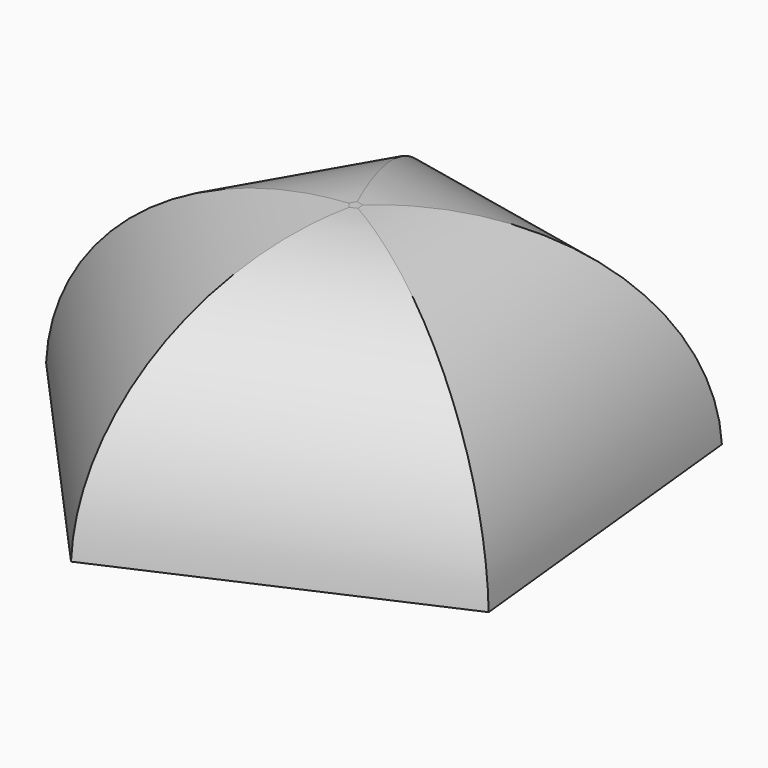
from build123d import *

# Parameters (mm, degrees)
F1_DEPTH    = 30
F2_T1_DEPTH = 201.5265861528
F2_T3_DEPTH = 201.5265861528
F2_T5_DEPTH = 201.5265861528
F2_T7_DEPTH = 201.5265861528
F2_T9_DEPTH = 201.5265861528


# Not quite as in the source:
# - a fillet or chamfer that OpenCascade refuses, or shapes differently, is made with other operations: its cross-section is extruded or revolved along the edge and cut away or added


with BuildPart() as f1:
    # F0 (on Top) → F1 (new body)
    with BuildSketch(Plane.XY):
        Polygon((-15.9371768066, 35.8527074811), (-39.0228095523, -4.0780599472), (-8.1802458333, -38.3730871366), (33.967139591, -19.6378121565), (29.1730926011, 26.2362517592), align=None)
    extrude(amount=F1_DEPTH)

    # F2: fillet of radius 31.1 on 5 edges, made by hand

    # F2_s2 → F2_t1 (cut)
    with BuildSketch(Plane(origin=(50.4334024594, 87.2336698068, 0), x_dir=(0, 0, 1), z_dir=(-0.5005136386, -0.8657286512, 0))):
        with BuildLine():
            ThreePointArc((0, 31.7420396575), (21.2765502256, 22.2601101881), (30, 0.6614991217))
            Line((30, 0.6614991217), (30, 31.7420396575))
            Line((30, 31.7420396575), (0, 31.7420396575))
        make_face()
    extrude(amount=F2_T1_DEPTH, mode=Mode.SUBTRACT)

    # F2_s4 → F2_t3 (cut)
    with BuildSketch(Plane(origin=(-67.379371666, 74.9217025, 0), x_dir=(0, 0, 1), z_dir=(0.6686896548, -0.7435416233, 0))):
        with BuildLine():
            ThreePointArc((0, 31.7420396575), (21.2765502256, 22.2601101881), (30, 0.6614991217))
            Line((30, 0.6614991217), (30, 31.7420396575))
            Line((30, 31.7420396575), (0, 31.7420396575))
        make_face()
    extrude(amount=F2_T3_DEPTH, mode=Mode.SUBTRACT)

    # F2_s6 → F2_t5 (cut)
    with BuildSketch(Plane(origin=(-92.0761442896, -40.9295111669, 0), x_dir=(0, 0, 1), z_dir=(0.9137865732, 0.406194656, 0))):
        with BuildLine():
            ThreePointArc((0, 31.7420396575), (21.2765502256, 22.2601101881), (30, 0.6614991217))
            Line((30, 0.6614991217), (30, 31.7420396575))
            Line((30, 31.7420396575), (0, 31.7420396575))
        make_face()
    extrude(amount=F2_T5_DEPTH, mode=Mode.SUBTRACT)

    # F2_s8 → F2_t7 (cut)
    with BuildSketch(Plane(origin=(10.473184942, -100.217531544, 0), x_dir=(0, 0, 1), z_dir=(-0.1039384941, 0.9945837267, 0))):
        with BuildLine():
            ThreePointArc((0, 31.7420396575), (21.2765502256, 22.2601101881), (30, 0.6614991217))
            Line((30, 0.6614991217), (30, 31.7420396575))
            Line((30, 31.7420396575), (0, 31.7420396575))
        make_face()
    extrude(amount=F2_T7_DEPTH, mode=Mode.SUBTRACT)

    # F2_s10 → F2_t9 (cut)
    with BuildSketch(Plane(origin=(98.5489285542, -21.0083295959, 0), x_dir=(0, 0, 1), z_dir=(-0.9780240953, 0.2084918918, 0))):
        with BuildLine():
            ThreePointArc((0, 31.7420396575), (21.2765502256, 22.2601101881), (30, 0.6614991217))
            Line((30, 0.6614991217), (30, 31.7420396575))
            Line((30, 31.7420396575), (0, 31.7420396575))
        make_face()
    extrude(amount=F2_T9_DEPTH, mode=Mode.SUBTRACT)


solid = f1.part
